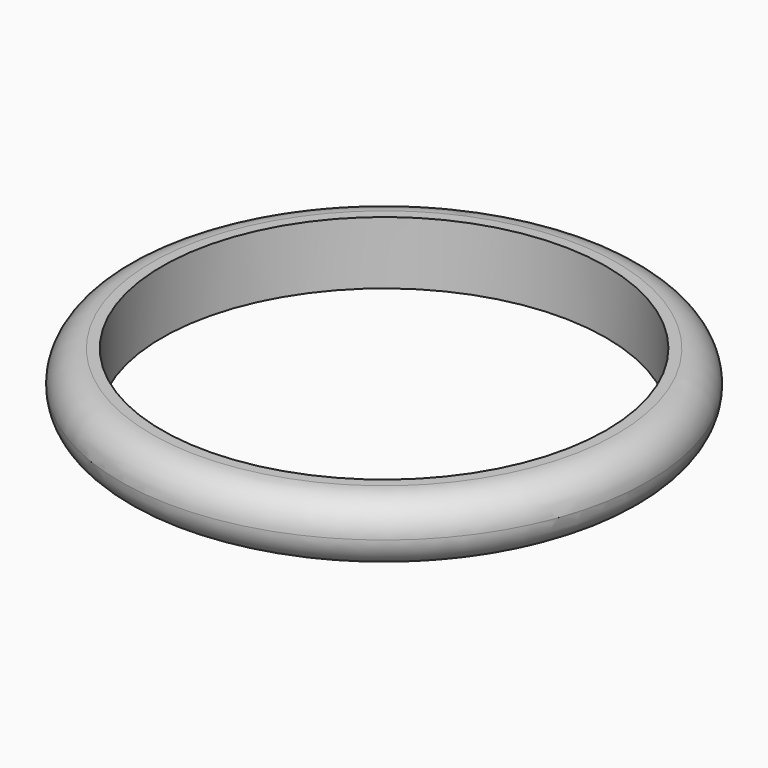
from build123d import *

# Parameters (mm, degrees)
F0_R     = 12.6
F0_R_2   = 10.6
F1_DEPTH = 3
F2_R     = 1.49999


# Not quite as in the source:
# - a fillet or chamfer is up to 0.001 mm smaller than in the source, because OpenCascade refuses the exact size


with BuildPart() as f1:
    # F0 (on Top) → F1 (new body)
    with BuildSketch(Plane.XY):
        Circle(F0_R)
        Circle(F0_R_2, mode=Mode.SUBTRACT)
    extrude(amount=F1_DEPTH)

    # F2 (radius 1.5 in the source; OpenCascade refuses exactly that, so slightly less here)
    f2_edges = [f1.edges().sort_by_distance(p)[0] for p in [
        (-12.6, 0, 3),
        (-12.6, 0, 0),
    ]]
    fillet(f2_edges, radius=F2_R)


solid = f1.part
